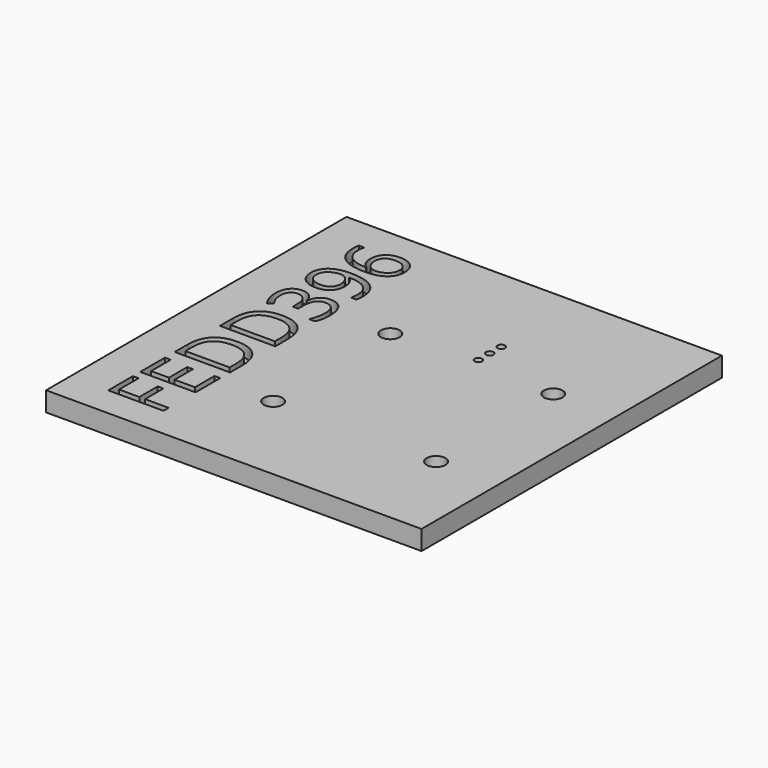
from build123d import *

# Parameters (mm, degrees)
F0_W         = 50
F0_H         = 50
F1_DEPTH     = 2.6
F2_TEXT_SIZE = 10.3248515069
F3_DEPTH     = 1.5
F4_R         = 1.25
F4_R_2       = 0.5
F5_DEPTH     = 2.6


# Not quite as in the source:
# - Text() gives the source's letters only with a copy of the font that has no kerning and outlines rounded to 1/6400 em; it was checked with that copy


with BuildPart() as f1:
    # F0 (on Top) → F1 (new body)
    with BuildSketch(Plane.XY):
        with Locations((-18.1587231159, 3.3350909071)):
            Rectangle(F0_W, F0_H)
    extrude(amount=F1_DEPTH)

    # F2 (on face) → F3 (cut)
    with BuildSketch(Plane.XY.offset(2.6)):
        with Locations(Location((-30.7248300309, -18.6649090929), (0, 0, 90))):
            Text('FEDD396', F2_TEXT_SIZE, font='Open Sans', text_align=(TextAlign.LEFT, TextAlign.BOTTOM))
    extrude(amount=-F3_DEPTH, mode=Mode.SUBTRACT)

    # F4 (on face) → F5 (cut, through all)
    with BuildSketch(Plane.XY.offset(2.6)):
        with Locations((-23.1587231159, -8.8684090929)):
            Circle(F4_R)
        with Locations((-23.1587231159, 10.6315909071)):
            Circle(F4_R)
        with Locations((-12.3087231159, 11.7265909071)):
            Circle(F4_R_2)
        with Locations((-12.3087231159, 13.6315909071)):
            Circle(F4_R_2)
        with Locations((-12.3087231159, 15.5365909071)):
            Circle(F4_R_2)
        with Locations((-1.4587231159, -8.8684090929)):
            Circle(F4_R)
        with Locations((-1.4587231159, 10.6315909071)):
            Circle(F4_R)
    extrude(amount=-F5_DEPTH, mode=Mode.SUBTRACT)


solid = f1.part
